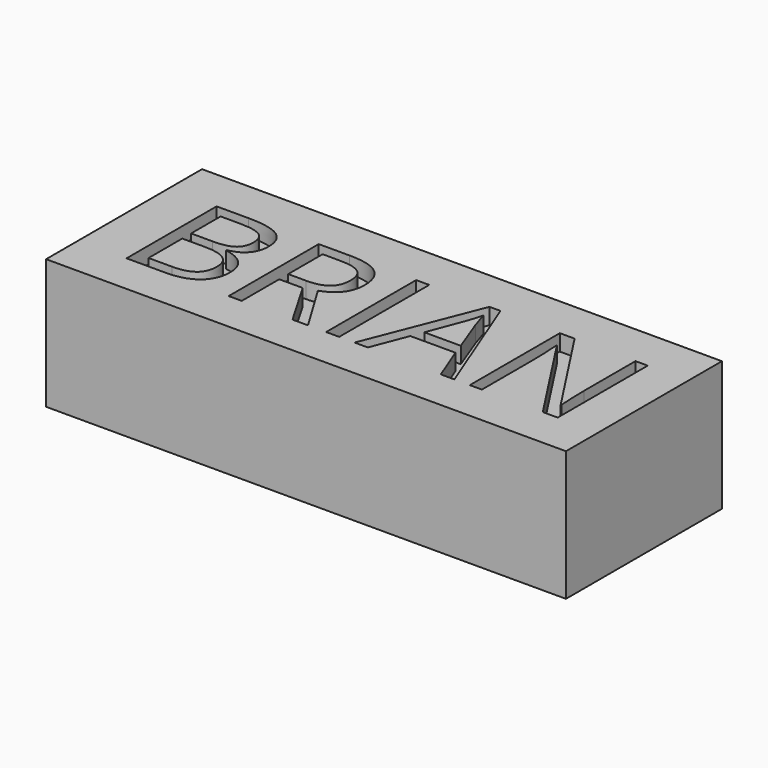
from build123d import *

# Parameters (mm, degrees)
F0_W         = 203.2
F0_H         = 76.2
F1_DEPTH     = 50.8
F2_TEXT_SIZE = 61.6100022
F3_DEPTH     = 6.35


# Not quite as in the source:
# - Text() gives the source's letters only with a copy of the font that has no kerning and outlines rounded to 1/6400 em; it was checked with that copy


with BuildPart() as f1:
    # F0 (on Top) → F1 (new body)
    with BuildSketch(Plane.XY):
        with Locations((101.6, 38.1)):
            Rectangle(F0_W, F0_H)
    extrude(amount=F1_DEPTH)

    # F2 (on face) → F3 (cut)
    with BuildSketch(Plane.XY.offset(50.8)):
        with Locations((12.7778142108, 15.7855842927)):
            Text('BRIAN', F2_TEXT_SIZE, font='Open Sans', text_align=(TextAlign.LEFT, TextAlign.BOTTOM))
    extrude(amount=-F3_DEPTH, mode=Mode.SUBTRACT)


solid = f1.part
